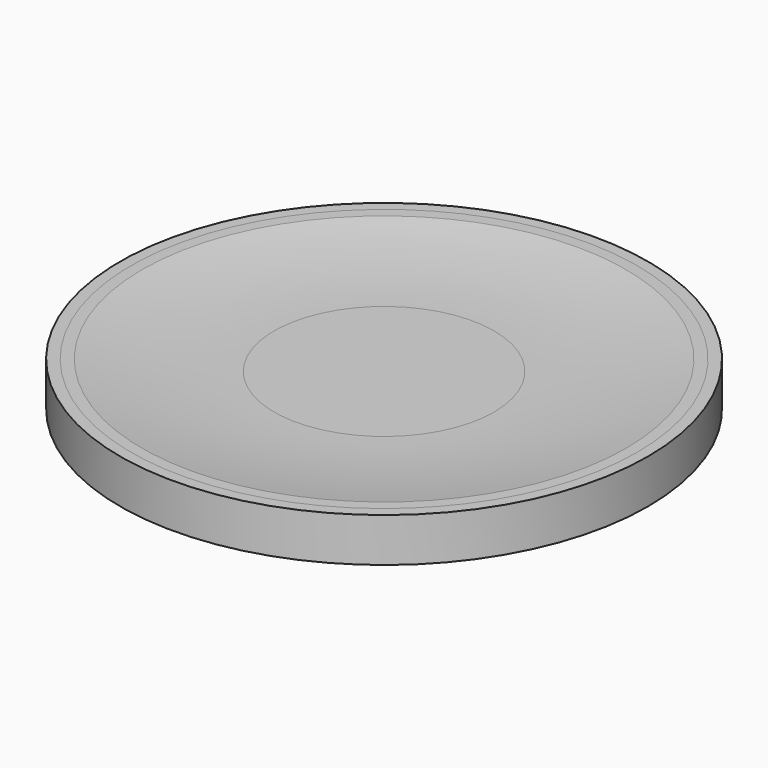
from build123d import *


# Not quite as in the source:
# - a feature of the source that left no trace in its solid (it failed there, or was rolled back) is left out
# - a feature names something its author has since deleted; it is built from what else it names


with BuildPart() as f1:
    # F0 (on Front) → F1 (revolve)
    with BuildSketch(Plane.XZ):
        Polygon((0, 5), (0, 0), (4, 0), (4, 3.5), (4.5, 4), (12, 4), (12, 6), (11.5, 6), (10.5, 5), align=None)
    revolve(axis=Axis((0, 0, 2.5), (0, 0, -1)))


with BuildPart() as f2:
    # F0 (on Front) → F2 (revolve)
    with BuildSketch(Plane.XZ):
        with BuildLine():
            Line((0, 5.5), (0, 5))
            Line((0, 5), (10.5, 5))
            Line((10.5, 5), (11.5, 6))
            Line((11.5, 6), (11, 6))
            ThreePointArc((11, 6), (8.0103986447, 5.6252162636), (5, 5.5))
            Line((5, 5.5), (0, 5.5))
        make_face()
    revolve(axis=Axis((0, 0, 2.5), (0, 0, -1)))


solid = Compound([f1.part, f2.part])
